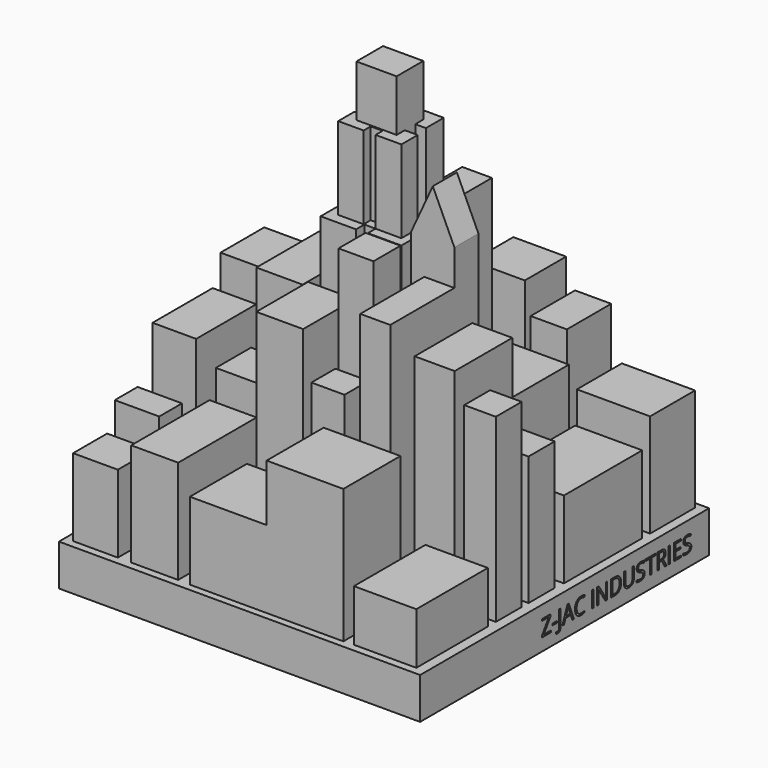
from build123d import *

# Parameters (mm, degrees)
F1_DEPTH      = 10.16
F2_W          = 19.3529091775
F2_H          = 13.062145561
F2_W_2        = 37.7717483789
F2_H_2        = 17.5461303443
F2_W_3        = 16.5024977177
F2_H_3        = 24.0809957031
F2_W_4        = 11.0106654465
F2_H_4        = 10.4658827186
F3_DEPTH      = 19.05
F4_W          = 11.5654263645
F4_H          = 24.1031181067
F4_W_2        = 10.9314583242
F4_H_2        = 7.015094161
F4_W_3        = 18.0117283016
F4_H_3        = 13.8405933976
F4_W_4        = 18.7701173127
F4_H_4        = 8.9393295348
F5_DEPTH      = 25.4
F6_W          = 11.1862337217
F6_H          = 10.8070378192
F6_W_2        = 17.4429386389
F6_H_2        = 12.7030108124
F6_W_3        = 8.0449385568
F6_H_3        = 8.057879284
F6_W_4        = 16.67467691
F6_H_4        = 19.1775755957
F7_DEPTH      = 31.75
F8_W          = 8.9110676199
F8_H          = 13.6509947479
F8_W_2        = 10.7418633997
F8_H_2        = 18.4857230633
F9_DEPTH      = 37.592
F10_W         = 10.55226475
F10_H         = 13.4613984264
F10_W_2       = 7.7734850347
F10_H_2       = 7.9630818218
F10_W_3       = 12.9874031991
F10_H_3       = 12.7030070871
F11_DEPTH     = 44.45
F12_W         = 11.3758305088
F12_H         = 19.7181045078
F13_DEPTH     = 48.26
F14_W         = 15.3573732823
F14_H         = 21.9932701439
F15_DEPTH     = 12.7
F16_W         = 16.8741479283
F16_H         = 9.5887877978
F16_W_2       = 9.859053418
F16_H_2       = 17.7273340523
F16_W_3       = 11.5224141628
F16_H_3       = 15.9261594526
F17_DEPTH     = 50.8
F18_W         = 5.4983170703
F18_H         = 5.7833152215
F18_W_2       = 4.2659351602
F18_H_2       = 5.2145229976
F18_W_3       = 6.4463026356
F18_H_3       = 5.0243246369
F19_DEPTH     = 63.5
F20_W         = 2.6543599088
F20_H         = 2.7491580695
F20_W_2       = 3.1757529359
F20_W_3       = 3.7919420283
F20_H_2       = 2.8439573944
F21_DEPTH     = 20.32
F22_W         = 9.9064516835
F22_H         = 8.2000775728
F23_DEPTH     = 12.7
F24_W         = 7.2994926013
F24_H         = 9.5887877978
F24_W_2       = 8.5972321685
F24_H_2       = 8.304010611
F25_DEPTH     = 66.04
F26_W         = 7.3942886665
F26_H         = 19.7181054391
F27_DEPTH     = 58.42
F28_W         = 10.6174396351
F28_H         = 7.3942891322
F29_DEPTH     = 20.32
F31_DEPTH     = 25.4
F32_W         = 8.1526774447
F32_H         = 7.3942914605
F33_DEPTH     = 40.64
F34_TEXT_SIZE = 5.6106438731
F35_DEPTH     = 2.54
F36_W         = 18.8858741894
F36_H         = 17.5461303443
F37_DEPTH     = 13.97


# Not quite as in the source:
# - Text() gives the source's letters only with a copy of the font that has no kerning and outlines rounded to 1/6400 em; it was checked with that copy


with BuildPart() as f1:
    # F0 (on Top) → F1 (new body)
    with BuildSketch(Plane.XY):
        Polygon((46.5250351965, 44.45), (0, 44.45), (-42.3749648035, 44.45), (-42.3749648035, -44.45), (46.5250351965, -44.45), align=None)
    extrude(amount=F1_DEPTH)

    # F2 (on face) → F3 (join)
    with BuildSketch(Plane.XY.offset(10.16)):
        with Locations((-31.2324184924, 36.5147236735)):
            Rectangle(F2_W, F2_H)
        with Locations((7.3634600267, -33.9467013255)):
            Rectangle(F2_W_2, F2_H_2)
        with Locations((36.0364029184, 14.6261657355)):
            Rectangle(F2_W_3, F2_H_3)
        with Locations((-34.8632689565, -37.3558998108)):
            Rectangle(F2_W_4, F2_H_4)
    extrude(amount=F3_DEPTH)

    # F4 (on face) → F5 (join)
    with BuildSketch(Plane.XY.offset(10.16)):
        with Locations((-20.286896266, -30.5372821167)):
            Rectangle(F4_W, F4_H)
        with Locations((-34.8236653954, -26.3540036976)):
            Rectangle(F4_W_2, F4_H_2)
        with Locations((35.2650722489, 36.0234603286)):
            Rectangle(F4_W_3, F4_H_3)
        with Locations((-30.9043359011, 22.1969988197)):
            Rectangle(F4_W_4, F4_H_4)
    extrude(amount=F5_DEPTH)

    # F6 (on face) → F7 (join)
    with BuildSketch(Plane.XY.offset(10.16)):
        with Locations((-20.2868958004, -11.3758293446)):
            Rectangle(F6_W, F6_H)
        with Locations((-10.3330459679, 36.5922516212)):
            Rectangle(F6_W_2, F6_H_2)
        with Locations((40.0588721968, -4.028939642)):
            Rectangle(F6_W_3, F6_H_3)
        with Locations((17.9119957611, 17.0778757893)):
            Rectangle(F6_W_4, F6_H_4)
    extrude(amount=F7_DEPTH)

    # F8 (on face) → F9 (join)
    with BuildSketch(Plane.XY.offset(10.16)):
        with Locations((19.3389104679, 35.9286610037)):
            Rectangle(F8_W, F8_H)
        with Locations((-34.7288679332, -9.2428615317)):
            Rectangle(F8_W_2, F8_H_2)
    extrude(amount=F9_DEPTH)

    # F10 (on face) → F11 (join)
    with BuildSketch(Plane.XY.offset(10.16)):
        with Locations((-34.6340686083, 8.9110664558)):
            Rectangle(F10_W, F10_H)
        with Locations((40.1945989579, -14.1249885783)):
            Rectangle(F10_W_2, F10_H_2)
        with Locations((6.4937015995, 36.0234575346)):
            Rectangle(F10_W_3, F10_H_3)
    extrude(amount=F11_DEPTH)

    # F12 (on face) → F13 (join)
    with BuildSketch(Plane.XY.offset(10.16)):
        with Locations((-20.3816941939, 5.7827134151)):
            Rectangle(F12_W, F12_H)
    extrude(amount=F13_DEPTH)

    # F14 (on face) → F15 (join)
    with BuildSketch(Plane.XY.offset(10.16)):
        with Locations((36.4026548341, -31.5679283813)):
            Rectangle(F14_W, F14_H)
    extrude(amount=F15_DEPTH)

    # F16 (on face) → F17 (join)
    with BuildSketch(Plane.XY.offset(10.16)):
        with Locations((-10.2382458863, 21.8722696882)):
            Rectangle(F16_W, F16_H)
        with Locations((28.7239709869, -8.8636670262)):
            Rectangle(F16_W_2, F16_H_2)
        with Locations((-5.7612070814, -14.3145846669)):
            Rectangle(F16_W_3, F16_H_3)
    extrude(amount=F17_DEPTH)

    # F18 (on face) → F19 (join)
    with BuildSketch(Plane.XY.offset(10.16)):
        Polygon((-9.1954618692, 7.6786847785), (-9.1954618692, 13.462), (-3.6971447989, 13.462), (-3.6971447989, 15.641765669), (-11.470627971, 15.641765669), (-11.470627971, 7.6786847785), align=None)
        with Locations((-6.4463033341, 10.5703423893)):
            Rectangle(F18_W, F18_H)
        Polygon((0, 13.462), (-3.6971447989, 13.462), (-3.6971447989, 7.6786847785), (-9.1954618692, 7.6786847785), (-9.1954618692, 5.0243246369), (-2.7491592336, 5.0243246369), (-2.7491592336, 0), (0, 0), (0, 5.0243246369), (4.2659351602, 5.0243246369), (4.2659351602, 8.2474770024), (0, 8.2474770024), align=None)
        Polygon((0, 15.641765669), (0, 13.462), (4.2659351602, 13.462), (4.2659351602, 8.2474770024), (7.6786838472, 8.2474770024), (7.6786838472, 15.641765669), align=None)
        with Locations((2.1329675801, 10.8547385012)):
            Rectangle(F18_W_2, F18_H_2)
        with Locations((-5.9723105514, 2.5121623185)):
            Rectangle(F18_W_3, F18_H_3)
        Polygon((-9.1954618692, 0), (-9.1954618692, 5.0243246369), (-11.470627971, 5.0243246369), (-11.470627971, -2.5595615152), (-2.7491592336, -2.5595615152), (-2.7491592336, 0), align=None)
        Polygon((8.2474751398, 5.0243246369), (4.2659351602, 5.0243246369), (4.2659351602, 0), (0, 0), (0, -2.3699644953), (8.2474751398, -2.3699644953), align=None)
        with Locations((2.1329675801, 2.5121623185)):
            Rectangle(F18_W_2, F18_H_3)
    extrude(amount=F19_DEPTH)

    # F20 (on face) → F21 (join)
    with BuildSketch(Plane.XY.offset(73.66)):
        Polygon((-4.0763388388, 13.7457931414), (-9.3850586563, 13.7457931414), (-9.3850586563, 8.2474770024), (-6.7306987476, 8.2474770024), (-6.7306987476, 10.9966350719), (-4.0763388388, 10.9966350719), align=None)
        Polygon((0, 10.9966350719), (-4.0763388388, 10.9966350719), (-4.0763388388, 8.2474770024), (-6.7306987476, 8.2474770024), (-6.7306987476, 5.0243246369), (-2.9387567192, 5.0243246369), (-2.9387567192, 2.1803672425), (0, 2.1803672425), (0, 5.0243246369), (3.1757529359, 5.0243246369), (3.1757529359, 8.2474770024), (0, 8.2474770024), align=None)
        with Locations((-5.4035187932, 9.6220560372)):
            Rectangle(F20_W, F20_H)
        with Locations((1.587876468, 9.6220560372)):
            Rectangle(F20_W_2, F20_H)
        Polygon((0, 13.7457931414), (0, 10.9966350719), (3.1757529359, 10.9966350719), (3.1757529359, 8.2474770024), (5.7827150449, 8.2474770024), (5.7827150449, 13.7457931414), align=None)
        Polygon((-6.7306987476, 2.1803672425), (-6.7306987476, 5.0243246369), (-9.1954618692, 5.0243246369), (-9.1954618692, 0), (-2.9387567192, 0), (-2.9387567192, 2.1803672425), align=None)
        with Locations((-4.8347277334, 3.6023459397)):
            Rectangle(F20_W_3, F20_H_2)
        with Locations((1.587876468, 3.6023459397)):
            Rectangle(F20_W_2, F20_H_2)
        Polygon((6.3515058719, 5.0243246369), (3.1757529359, 5.0243246369), (3.1757529359, 2.1803672425), (0, 2.1803672425), (0, 0), (6.3515058719, 0), align=None)
    extrude(amount=F21_DEPTH)

    # F22 (on face) → F23 (join)
    with BuildSketch(Plane.XY.offset(93.98)):
        with Locations((-1.7774729058, 6.6122011049)):
            Rectangle(F22_W, F22_H)
    extrude(amount=F23_DEPTH)

    # F24 (on face) → F25 (join)
    with BuildSketch(Plane.XY.offset(10.16)):
        with Locations((3.6497463007, 21.8722696882)):
            Rectangle(F24_W, F24_H)
        with Locations((6.9108485477, -10.5035102461)):
            Rectangle(F24_W_2, F24_H_2)
    extrude(amount=F25_DEPTH)

    # F26 (on face) → F27 (join)
    with BuildSketch(Plane.XY.offset(10.16)):
        Polygon((21.1400836706, 5.2139218897), (10.5226440355, 5.2139218897), (10.5226440355, -2.1803672425), (13.7457950041, -2.1803672425), (21.1400836706, -2.1803672425), align=None)
        with Locations((17.4429393373, -12.0394199621)):
            Rectangle(F26_W, F26_H)
    extrude(amount=F27_DEPTH)

    # F28 (on face) → F29 (join)
    with BuildSketch(Plane.XY.offset(68.58)):
        with Locations((15.8313638531, 1.5167773236)):
            Rectangle(F28_W, F28_H)
    extrude(amount=F29_DEPTH)

    # F30 (on face) → F31 (cut)
    with BuildSketch(Plane.XZ.offset(2.1803672425)):
        Polygon((10.5226440355, 77.3627778951), (15.8313638531, 88.9), (10.5226440355, 88.9), align=None)
        Polygon((21.1400836706, 88.9), (15.8313638531, 88.9), (21.1400836706, 77.3627778951), align=None)
    extrude(amount=-F31_DEPTH, mode=Mode.SUBTRACT)

    # F32 (on face) → F33 (join)
    with BuildSketch(Plane.XY.offset(10.16)):
        with Locations((7.0150956744, -19.7181049734)):
            Rectangle(F32_W, F32_H)
    extrude(amount=F33_DEPTH)

    # F34 (on face) → F35 (cut)
    with BuildSketch(Plane.YZ.offset(46.5250351965)):
        with Locations((-7.1966564283, 3.0465538148)):
            Text('Z-JAC INDUSTRIES', F34_TEXT_SIZE, font='Open Sans', text_align=(TextAlign.LEFT, TextAlign.BOTTOM))
    extrude(amount=-F35_DEPTH, mode=Mode.SUBTRACT)

    # F36 (on face) → F37 (join)
    with BuildSketch(Plane.XY.offset(29.21)):
        with Locations((16.8063971214, -33.9467013255)):
            Rectangle(F36_W, F36_H)
    extrude(amount=F37_DEPTH)


solid = f1.part
